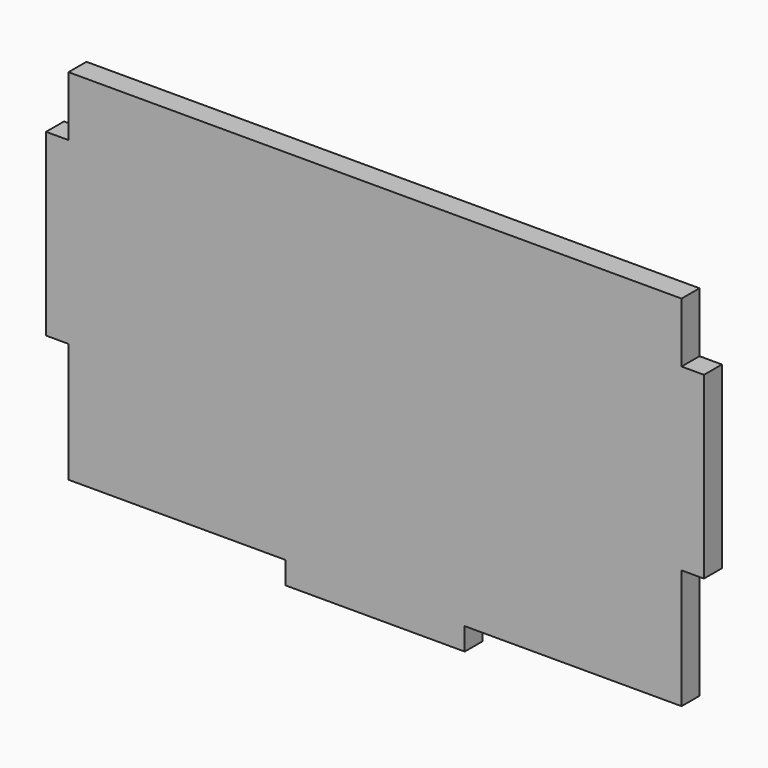
from build123d import *

# Parameters (mm, degrees)
F0_W     = 19.05
F0_H     = 152.4
F0_W_2   = 152.4
F0_H_2   = 19.05
F1_DEPTH = 19.05


# Not quite as in the source:
# - a feature names something its author has since deleted; it is built from what else it names


with BuildPart() as f1:
    # F0 (on Front) → F1 (new body)
    with BuildSketch(Plane.XZ):
        Polygon((-388.9506477541, -103.6229937509), (-204.8006477541, -103.6229937509), (-204.8006477541, -2.0229937509), (-204.8006477541, 150.3770062491), (-204.8006477541, 201.1770062491), (-725.5006477541, 201.1770062491), (-725.5006477541, 150.3770062491), (-725.5006477541, -2.0229937509), (-725.5006477541, -103.6229937509), (-541.3506477541, -103.6229937509), align=None)
        with Locations((-735.0256477541, 74.1770062491)):
            Rectangle(F0_W, F0_H)
        with Locations((-195.2756477541, 74.1770062491)):
            Rectangle(F0_W, F0_H)
        with Locations((-465.1506477541, -113.1479937509)):
            Rectangle(F0_W_2, F0_H_2)
    extrude(amount=F1_DEPTH)


solid = f1.part
